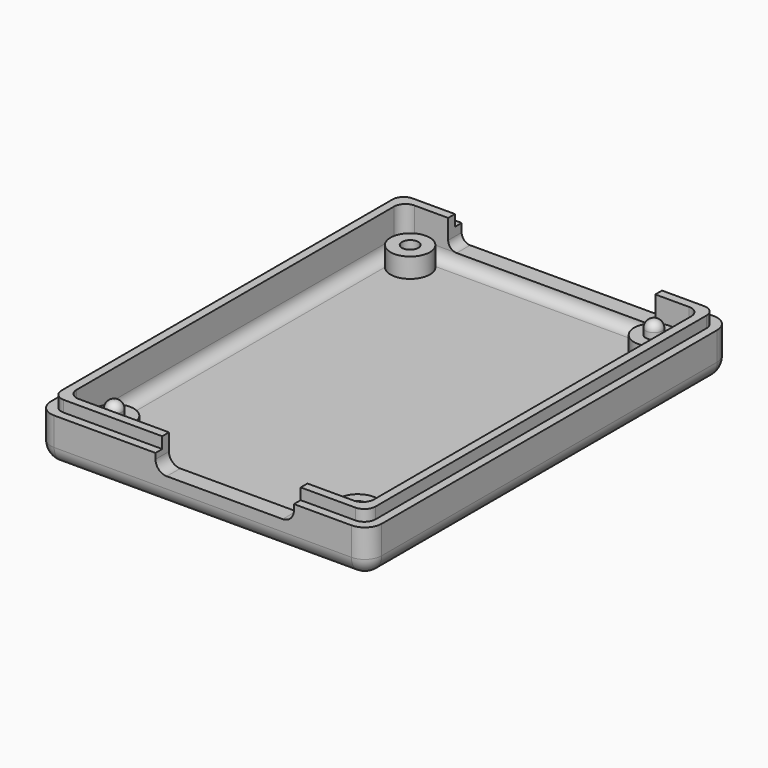
from build123d import *

# Parameters (mm, degrees)
F0_W          = 58.8
F0_H          = 80.5
F1_DEPTH      = 8
F2_W          = 52.8
F2_H          = 74.5
F3_DEPTH      = 5
F5_R          = 3.5
F6_DEPTH      = 3.5
F9_R          = 1.45
F7_R          = 1.45
F11_DEPTH     = 6.501
F8_R          = 1.45
F12_DEPTH     = 2.5
F10_R         = 1.45
F13_R         = 1.4
F14_W         = 36.8
F14_H         = 3
F15_DEPTH     = 3
F16_W         = 24.6
F16_H         = 3
F17_DEPTH     = 3
F20_DEPTH     = 2
F21_R         = 3
F22_T1_DEPTH  = 5
F22_T3_DEPTH  = 70.5
F22_T5_DEPTH  = 48.8
F22_S9_W      = 2
F22_S9_H      = 2
F22_T10_DEPTH = 2
F22_S15_W     = 2
F22_S15_H     = 2
F22_T16_DEPTH = 2
F22_S21_W     = 2
F22_S21_H     = 2
F22_T22_DEPTH = 2
F22_S27_W     = 2
F22_S27_H     = 2
F22_T28_DEPTH = 2
F23_R         = 2
F24_R         = 1.5
F25_R         = 2
F26_R         = 2.75
F27_DEPTH     = 1.6


# Not quite as in the source:
# - a fillet or chamfer that OpenCascade refuses, or shapes differently, is made with other operations: its cross-section is extruded or revolved along the edge and cut away or added


with BuildPart() as f1:
    # F0 (on Top) → F1 (new body)
    with BuildSketch(Plane.XY):
        with Locations((29.4, 40.25)):
            Rectangle(F0_W, F0_H)
    extrude(amount=F1_DEPTH)

    # F2 (on face) → F3 (cut)
    with BuildSketch(Plane.XY.offset(8)):
        with Locations((29.4, 40.25)):
            Rectangle(F2_W, F2_H)
    extrude(amount=-F3_DEPTH, mode=Mode.SUBTRACT)

    # F5 (on face) → F6 (join)
    with BuildSketch(Plane.XY.offset(3)):
        with Locations((7.75, 7.375)):
            Circle(F5_R)
        with Locations((7.75, 73.125)):
            Circle(F5_R)
        with Locations((51.05, 73.125)):
            Circle(F5_R)
        with Locations((51.05, 7.375)):
            Circle(F5_R)
    extrude(amount=F6_DEPTH)

    # F9 (on face) + F7 (on face) → F11 (cut, through all)
    with BuildSketch(Plane.XY.offset(6.5)):
        with Locations((7.75, 73.125)):
            Circle(F9_R)
    with BuildSketch(Plane.XY.offset(6.5)):
        with Locations((51.05, 7.375)):
            Circle(F7_R)
    extrude(amount=-F11_DEPTH, mode=Mode.SUBTRACT)

    # F8 (on face) → F12 (join)
    with BuildSketch(Plane.XY.offset(6.5)):
        with Locations((51.05, 73.125)):
            Circle(F8_R)
    extrude(amount=F12_DEPTH)

    # F10 (on face) → F12, piece 2 (join)
    with BuildSketch(Plane.XY.offset(6.5)):
        with Locations((7.75, 7.375)):
            Circle(F10_R)
    extrude(amount=F12_DEPTH)

    # F13
    f13_edges = [f1.edges().sort_by_distance(p)[0] for p in [
        (6.3, 7.375, 9),
        (49.6, 73.125, 9),
    ]]
    fillet(f13_edges, radius=F13_R)

    # F14 (on face) → F15 (cut)
    with BuildSketch(Plane.XY.offset(8)):
        with Locations((29.4, 79)):
            Rectangle(F14_W, F14_H)
    extrude(amount=-F15_DEPTH, mode=Mode.SUBTRACT)

    # F16 (on face) → F17 (cut)
    with BuildSketch(Plane.XY.offset(8)):
        with Locations((33.3, 1.5)):
            Rectangle(F16_W, F16_H)
    extrude(amount=-F17_DEPTH, mode=Mode.SUBTRACT)

    # F18 (on face) → F20 (join)
    with BuildSketch(Plane.XY.offset(8)):
        Polygon((47.8, 79), (47.8, 77.5), (55.8, 77.5), (55.8, 3), (45.6, 3), (45.6, 1.5), (57.3, 1.5), (57.3, 79), align=None)
    extrude(amount=F20_DEPTH)

    # F19 (on face) → F20, piece 2 (join)
    with BuildSketch(Plane.XY.offset(8)):
        Polygon((1.5, 1.5), (21, 1.5), (21, 3), (3, 3), (3, 77.5), (11, 77.5), (11, 79), (1.5, 79), align=None)
    extrude(amount=F20_DEPTH)

    # F21
    f21_edges = [f1.edges().sort_by_distance(p)[0] for p in [
        (0, 0, 4),
        (29.4, 0, 0),
        (58.8, 0, 4),
        (0, 40.25, 0),
        (0, 80.5, 4),
        (29.4, 80.5, 0),
        (58.8, 80.5, 4),
        (58.8, 40.25, 0),
    ]]
    fillet(f21_edges, radius=F21_R)

    # F22: fillet of radius 2 on 8 edges, made by hand

    # F22_s2 → F22_t1 (join)
    with BuildSketch(Plane.XY.offset(5)):
        with BuildLine():
            ThreePointArc((53.8, 3), (55.2142135624, 3.5857864376), (55.8, 5))
            Line((55.8, 5), (55.8, 3))
            Line((55.8, 3), (53.8, 3))
        make_face()
        with BuildLine():
            ThreePointArc((5, 3), (3.5857864376, 3.5857864376), (3, 5))
            Line((3, 5), (3, 3))
            Line((3, 3), (5, 3))
        make_face()
        with BuildLine():
            ThreePointArc((5, 77.5), (3.5857864376, 76.9142135624), (3, 75.5))
            Line((3, 75.5), (3, 77.5))
            Line((3, 77.5), (5, 77.5))
        make_face()
        with BuildLine():
            ThreePointArc((53.8, 77.5), (55.2142135624, 76.9142135624), (55.8, 75.5))
            Line((55.8, 75.5), (55.8, 77.5))
            Line((55.8, 77.5), (53.8, 77.5))
        make_face()
    extrude(amount=F22_T1_DEPTH)

    # F22_s4 → F22_t3 (join)
    with BuildSketch(Plane.XZ.offset(-75.5)):
        with BuildLine():
            ThreePointArc((53.8, 3), (55.2142135624, 3.5857864376), (55.8, 5))
            Line((55.8, 5), (55.8, 3))
            Line((55.8, 3), (53.8, 3))
        make_face()
        with BuildLine():
            ThreePointArc((5, 3), (3.5857864376, 3.5857864376), (3, 5))
            Line((3, 5), (3, 3))
            Line((3, 3), (5, 3))
        make_face()
    extrude(amount=F22_T3_DEPTH)

    # F22_s6 → F22_t5 (join)
    with BuildSketch(Plane.YZ.offset(5)):
        with BuildLine():
            ThreePointArc((3, 5), (3.5857864376, 3.5857864376), (5, 3))
            Line((5, 3), (3, 3))
            Line((3, 3), (3, 5))
        make_face()
        with BuildLine():
            ThreePointArc((77.5, 5), (76.9142135624, 3.5857864376), (75.5, 3))
            Line((75.5, 3), (77.5, 3))
            Line((77.5, 3), (77.5, 5))
        make_face()
    extrude(amount=F22_T5_DEPTH)


with BuildPart() as f22_tool8:
    # F22_s9 → F22_t10 (new body)
    with BuildSketch(Plane.XY.offset(5)):
        with Locations((54.8, 4)):
            Rectangle(F22_S9_W, F22_S9_H)
    extrude(amount=-F22_T10_DEPTH)

    # F22_s11 → F22_t12 (revolve, cut)
    with BuildSketch(Plane(origin=(53.8, 5, 5), x_dir=(-0.7071067812, 0.7071067812, 0), z_dir=(-0.7071067812, -0.7071067812, 0))):
        with BuildLine():
            ThreePointArc((0, -2), (2, 0), (0, 2))
            Line((0, 2), (0, -2))
        make_face()
    revolve(axis=Axis((53.8, 5, 5), (0, 0, -1)), mode=Mode.SUBTRACT)


with BuildPart() as f1_1:
    add(f1.part)

    # F22_t7: union F22_tool8
    add(f22_tool8.part)


with BuildPart() as f22_tool14:
    # F22_s15 → F22_t16 (new body)
    with BuildSketch(Plane.XY.offset(5)):
        with Locations((4, 4)):
            Rectangle(F22_S15_W, F22_S15_H)
    extrude(amount=-F22_T16_DEPTH)

    # F22_s17 → F22_t18 (revolve, cut)
    with BuildSketch(Plane(origin=(5, 5, 5), x_dir=(0.7071067812, 0.7071067812, 0), z_dir=(-0.7071067812, 0.7071067812, 0))):
        with BuildLine():
            ThreePointArc((0, -2), (2, 0), (0, 2))
            Line((0, 2), (0, -2))
        make_face()
    revolve(axis=Axis((5, 5, 5), (0, 0, -1)), mode=Mode.SUBTRACT)


with BuildPart() as f1_2:
    add(f1_1.part)

    # F22_t13: union F22_tool14
    add(f22_tool14.part)


with BuildPart() as f22_tool20:
    # F22_s21 → F22_t22 (new body)
    with BuildSketch(Plane.XZ.offset(-75.5)):
        with Locations((4, 4)):
            Rectangle(F22_S21_W, F22_S21_H)
    extrude(amount=-F22_T22_DEPTH)

    # F22_s23 → F22_t24 (revolve, cut)
    with BuildSketch(Plane(origin=(5, 75.5, 5), x_dir=(0.7071067812, 0, 0.7071067812), z_dir=(-0.7071067812, 0, 0.7071067812))):
        with BuildLine():
            ThreePointArc((0, -2), (2, 0), (0, 2))
            Line((0, 2), (0, -2))
        make_face()
    revolve(axis=Axis((5, 75.5, 5), (0, 1, 0)), mode=Mode.SUBTRACT)


with BuildPart() as f1_3:
    add(f1_2.part)

    # F22_t19: union F22_tool20
    add(f22_tool20.part)


with BuildPart() as f22_tool26:
    # F22_s27 → F22_t28 (new body)
    with BuildSketch(Plane.XZ.offset(-75.5)):
        with Locations((54.8, 4)):
            Rectangle(F22_S27_W, F22_S27_H)
    extrude(amount=-F22_T28_DEPTH)

    # F22_s29 → F22_t30 (revolve, cut)
    with BuildSketch(Plane(origin=(53.8, 75.5, 5), x_dir=(-0.7071067812, 0, 0.7071067812), z_dir=(-0.7071067812, 0, -0.7071067812))):
        with BuildLine():
            ThreePointArc((0, -2), (2, 0), (0, 2))
            Line((0, 2), (0, -2))
        make_face()
    revolve(axis=Axis((53.8, 75.5, 5), (0, 1, 0)), mode=Mode.SUBTRACT)


with BuildPart() as f1_4:
    add(f1_3.part)

    # F22_t25: union F22_tool26
    add(f22_tool26.part)

    # F23
    f23_edges = [f1_4.edges().sort_by_distance(p)[0] for p in [
        (57.3, 79, 9),
        (1.5, 79, 9),
        (1.5, 1.5, 9),
        (57.3, 1.5, 9),
    ]]
    fillet(f23_edges, radius=F23_R)

    # F24
    f24_edges = [f1_4.edges().sort_by_distance(p)[0] for p in [
        (11, 79, 5),
        (47.8, 79, 5),
    ]]
    fillet(f24_edges, radius=F24_R)

    # F25
    f25_edges = [f1_4.edges().sort_by_distance(p)[0] for p in [
        (21, 1.5, 5),
        (45.6, 1.5, 5),
    ]]
    fillet(f25_edges, radius=F25_R)

    # F26 (on face) → F27 (cut)
    with BuildSketch(Plane(origin=(0, 0, 0), x_dir=(1, 0, 0), z_dir=(0, 0, -1))):
        with Locations((51.05, -7.375)):
            Circle(F26_R)
        with Locations((7.75, -73.125)):
            Circle(F26_R)
    extrude(amount=-F27_DEPTH, mode=Mode.SUBTRACT)


solid = f1_4.part
